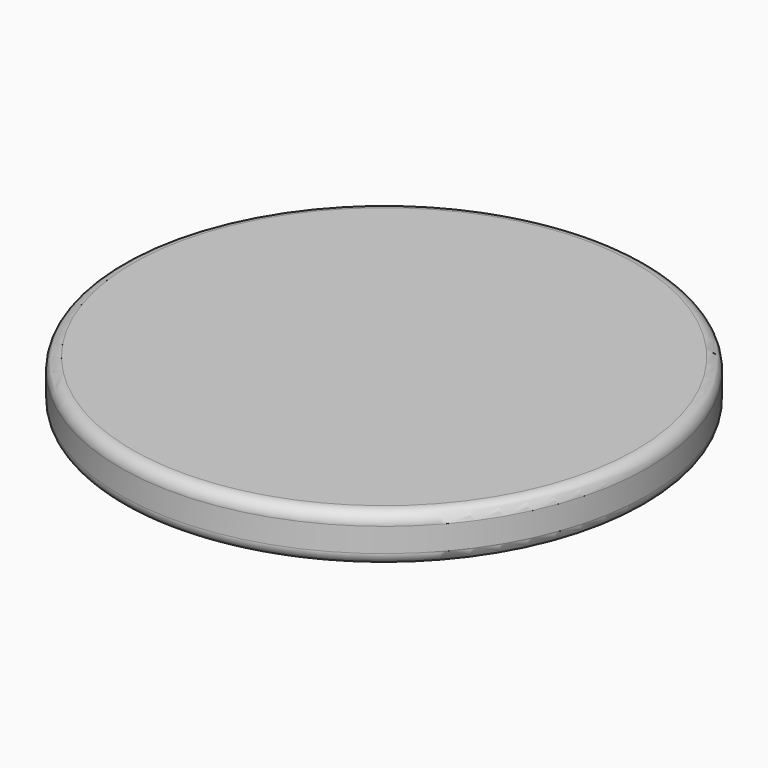
from build123d import *

# Parameters (mm, degrees)
F0_W   = 4.1
F0_H   = 0.4
F0_W_2 = 1.9
F0_H_2 = 2.8
F2_R   = 0.5


with BuildPart() as f1:
    # F0 (on Front) → F1 (revolve)
    with BuildSketch(Plane.XZ):
        Polygon((0, 2), (0, 0), (4.1, 0), (6, 0), (11, 0), (11, 2), align=None)
        with Locations((2.05, -0.2)):
            Rectangle(F0_W, F0_H)
        with Locations((5.05, -0.2)):
            Rectangle(F0_W_2, F0_H)
        with Locations((2.05, -1.8)):
            Rectangle(F0_W, F0_H_2)
    revolve(axis=Axis((0, 0, 1), (0, 0, 1)))

    # F2
    f2_edges = [f1.edges().sort_by_distance(p)[0] for p in [
        (-11, 0, 0),
        (-11, 0, 2),
    ]]
    fillet(f2_edges, radius=F2_R)


solid = f1.part
